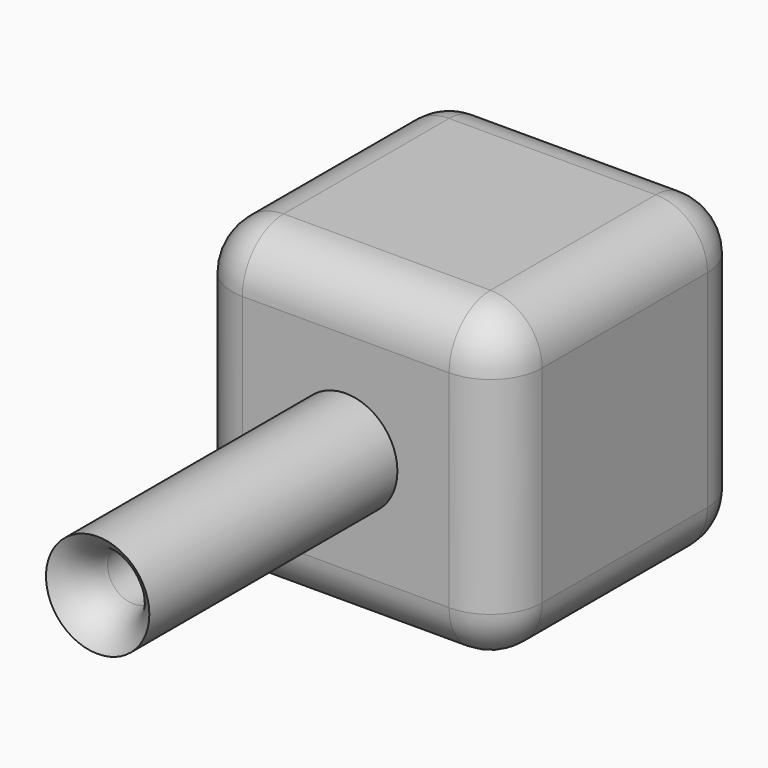
from build123d import *

# Parameters (mm, degrees)
F0_W         = 30
F0_H         = 30
F1_DEPTH     = 30
F2_R         = 5
F3_DEPTH     = 30
F4_R         = 2.5001325449
F5_DEPTH     = 60.001
F6_T1_DEPTH  = 20
F6_T3_DEPTH  = 20
F6_T5_DEPTH  = 20
F6_S9_W      = 5.1
F6_S9_H      = 5.1
F6_T10_DEPTH = 5.1
F6_S15_W     = 5.1
F6_S15_H     = 5.1
F6_T16_DEPTH = 5.1
F6_S21_W     = 5.1
F6_S21_H     = 5.1
F6_T22_DEPTH = 5.1
F6_S27_W     = 5.1
F6_S27_H     = 5.1
F6_T28_DEPTH = 5.1
F6_S33_W     = 5.1
F6_S33_H     = 5.1
F6_T34_DEPTH = 5.1
F6_S39_W     = 5.1
F6_S39_H     = 5.1
F6_T40_DEPTH = 5.1
F6_S45_W     = 5.1
F6_S45_H     = 5.1
F6_T46_DEPTH = 5.1
F6_S51_W     = 5.1
F6_S51_H     = 5.1
F6_T52_DEPTH = 5.1


# Not quite as in the source:
# - a fillet or chamfer that OpenCascade refuses, or shapes differently, is made with other operations: its cross-section is extruded or revolved along the edge and cut away or added


with BuildPart() as f1:
    # F0 (on Front) → F1 (new body)
    with BuildSketch(Plane.XZ):
        Rectangle(F0_W, F0_H)
    extrude(amount=F1_DEPTH)

    # F2 (on face) → F3 (join)
    with BuildSketch(Plane.XZ.offset(30)):
        Circle(F2_R)
    extrude(amount=F3_DEPTH)

    # F4 (on face) → F5 (cut, through all)
    with BuildSketch(Plane.XZ.offset(60)):
        Circle(F4_R)
    extrude(amount=-F5_DEPTH, mode=Mode.SUBTRACT)

    # F6: fillet of radius 5 on 13 edges, made by hand

    # F6_s2 → F6_t1 (cut)
    with BuildSketch(Plane.XZ.offset(5)):
        with BuildLine():
            ThreePointArc((10, 15), (13.5355339059, 13.5355339059), (15, 10))
            Line((15, 10), (15, 15))
            Line((15, 15), (10, 15))
        make_face()
        with BuildLine():
            ThreePointArc((-10, 15), (-13.5355339059, 13.5355339059), (-15, 10))
            Line((-15, 10), (-15, 15))
            Line((-15, 15), (-10, 15))
        make_face()
        with BuildLine():
            ThreePointArc((-15, -10), (-13.5355339059, -13.5355339059), (-10, -15))
            Line((-10, -15), (-15, -15))
            Line((-15, -15), (-15, -10))
        make_face()
        with BuildLine():
            ThreePointArc((15, -10), (13.5355339059, -13.5355339059), (10, -15))
            Line((10, -15), (15, -15))
            Line((15, -15), (15, -10))
        make_face()
    extrude(amount=F6_T1_DEPTH, mode=Mode.SUBTRACT)

    # F6_s4 → F6_t3 (cut)
    with BuildSketch(Plane.YZ.offset(-10)):
        with BuildLine():
            ThreePointArc((-25, 15), (-28.5355339059, 13.5355339059), (-30, 10))
            Line((-30, 10), (-30, 15))
            Line((-30, 15), (-25, 15))
        make_face()
        with BuildLine():
            ThreePointArc((-5, 15), (-1.4644660941, 13.5355339059), (0, 10))
            Line((0, 10), (0, 15))
            Line((0, 15), (-5, 15))
        make_face()
        with BuildLine():
            ThreePointArc((-30, -10), (-28.5355339059, -13.5355339059), (-25, -15))
            Line((-25, -15), (-30, -15))
            Line((-30, -15), (-30, -10))
        make_face()
        with BuildLine():
            ThreePointArc((0, -10), (-1.4644660941, -13.5355339059), (-5, -15))
            Line((-5, -15), (0, -15))
            Line((0, -15), (0, -10))
        make_face()
    extrude(amount=F6_T3_DEPTH, mode=Mode.SUBTRACT)

    # F6_s6 → F6_t5 (cut)
    with BuildSketch(Plane.XY.offset(-10)):
        with BuildLine():
            ThreePointArc((-15, -5), (-13.5355339059, -1.4644660941), (-10, 0))
            Line((-10, 0), (-15, 0))
            Line((-15, 0), (-15, -5))
        make_face()
        with BuildLine():
            ThreePointArc((-15, -25), (-13.5355339059, -28.5355339059), (-10, -30))
            Line((-10, -30), (-15, -30))
            Line((-15, -30), (-15, -25))
        make_face()
        with BuildLine():
            ThreePointArc((15, -5), (13.5355339059, -1.4644660941), (10, 0))
            Line((10, 0), (15, 0))
            Line((15, 0), (15, -5))
        make_face()
        with BuildLine():
            ThreePointArc((15, -25), (13.5355339059, -28.5355339059), (10, -30))
            Line((10, -30), (15, -30))
            Line((15, -30), (15, -25))
        make_face()
    extrude(amount=F6_T5_DEPTH, mode=Mode.SUBTRACT)


with BuildPart() as f6_tool8:
    # F6_s9 → F6_t10 (new body)
    with BuildSketch(Plane.XY.offset(10)):
        with Locations((12.55, -2.45)):
            Rectangle(F6_S9_W, F6_S9_H)
    extrude(amount=F6_T10_DEPTH)

    # F6_s11 → F6_t12 (revolve, cut)
    with BuildSketch(Plane(origin=(10, -5, 10), x_dir=(-0.7071067812, -0.7071067812, 0), z_dir=(-0.7071067812, 0.7071067812, 0))):
        with BuildLine():
            ThreePointArc((0, -5), (5, 0), (0, 5))
            Line((0, 5), (0, -5))
        make_face()
    revolve(axis=Axis((10, -5, 10), (0, 0, 1)), mode=Mode.SUBTRACT)


with BuildPart() as f1_1:
    add(f1.part)

    # F6_t7: cut F6_tool8
    add(f6_tool8.part, mode=Mode.SUBTRACT)


with BuildPart() as f6_tool14:
    # F6_s15 → F6_t16 (new body)
    with BuildSketch(Plane.XY.offset(10)):
        with Locations((12.55, -27.55)):
            Rectangle(F6_S15_W, F6_S15_H)
    extrude(amount=F6_T16_DEPTH)

    # F6_s17 → F6_t18 (revolve, cut)
    with BuildSketch(Plane(origin=(10, -25, 10), x_dir=(-0.7071067812, 0.7071067812, 0), z_dir=(0.7071067812, 0.7071067812, 0))):
        with BuildLine():
            ThreePointArc((0, -5), (5, 0), (0, 5))
            Line((0, 5), (0, -5))
        make_face()
    revolve(axis=Axis((10, -25, 10), (0, 0, 1)), mode=Mode.SUBTRACT)


with BuildPart() as f1_2:
    add(f1_1.part)

    # F6_t13: cut F6_tool14
    add(f6_tool14.part, mode=Mode.SUBTRACT)


with BuildPart() as f6_tool20:
    # F6_s21 → F6_t22 (new body)
    with BuildSketch(Plane.XY.offset(10)):
        with Locations((-12.55, -2.45)):
            Rectangle(F6_S21_W, F6_S21_H)
    extrude(amount=F6_T22_DEPTH)

    # F6_s23 → F6_t24 (revolve, cut)
    with BuildSketch(Plane(origin=(-10, -5, 10), x_dir=(0.7071067812, -0.7071067812, 0), z_dir=(-0.7071067812, -0.7071067812, 0))):
        with BuildLine():
            ThreePointArc((0, -5), (5, 0), (0, 5))
            Line((0, 5), (0, -5))
        make_face()
    revolve(axis=Axis((-10, -5, 10), (0, 0, 1)), mode=Mode.SUBTRACT)


with BuildPart() as f1_3:
    add(f1_2.part)

    # F6_t19: cut F6_tool20
    add(f6_tool20.part, mode=Mode.SUBTRACT)


with BuildPart() as f6_tool26:
    # F6_s27 → F6_t28 (new body)
    with BuildSketch(Plane.XY.offset(10)):
        with Locations((-12.55, -27.55)):
            Rectangle(F6_S27_W, F6_S27_H)
    extrude(amount=F6_T28_DEPTH)

    # F6_s29 → F6_t30 (revolve, cut)
    with BuildSketch(Plane(origin=(-10, -25, 10), x_dir=(0.7071067812, 0.7071067812, 0), z_dir=(0.7071067812, -0.7071067812, 0))):
        with BuildLine():
            ThreePointArc((0, -5), (5, 0), (0, 5))
            Line((0, 5), (0, -5))
        make_face()
    revolve(axis=Axis((-10, -25, 10), (0, 0, 1)), mode=Mode.SUBTRACT)


with BuildPart() as f1_4:
    add(f1_3.part)

    # F6_t25: cut F6_tool26
    add(f6_tool26.part, mode=Mode.SUBTRACT)


with BuildPart() as f6_tool32:
    # F6_s33 → F6_t34 (new body)
    with BuildSketch(Plane.YZ.offset(-10)):
        with Locations((-27.55, -12.55)):
            Rectangle(F6_S33_W, F6_S33_H)
    extrude(amount=-F6_T34_DEPTH)

    # F6_s35 → F6_t36 (revolve, cut)
    with BuildSketch(Plane(origin=(-10, -25, -10), x_dir=(0, 0.7071067812, 0.7071067812), z_dir=(0, -0.7071067812, 0.7071067812))):
        with BuildLine():
            ThreePointArc((0, -5), (5, 0), (0, 5))
            Line((0, 5), (0, -5))
        make_face()
    revolve(axis=Axis((-10, -25, -10), (-1, 0, 0)), mode=Mode.SUBTRACT)


with BuildPart() as f1_5:
    add(f1_4.part)

    # F6_t31: cut F6_tool32
    add(f6_tool32.part, mode=Mode.SUBTRACT)


with BuildPart() as f6_tool38:
    # F6_s39 → F6_t40 (new body)
    with BuildSketch(Plane.YZ.offset(10)):
        with Locations((-27.55, -12.55)):
            Rectangle(F6_S39_W, F6_S39_H)
    extrude(amount=F6_T40_DEPTH)

    # F6_s41 → F6_t42 (revolve, cut)
    with BuildSketch(Plane(origin=(10, -25, -10), x_dir=(0, 0.7071067812, 0.7071067812), z_dir=(0, 0.7071067812, -0.7071067812))):
        with BuildLine():
            ThreePointArc((0, -5), (5, 0), (0, 5))
            Line((0, 5), (0, -5))
        make_face()
    revolve(axis=Axis((10, -25, -10), (1, 0, 0)), mode=Mode.SUBTRACT)


with BuildPart() as f1_6:
    add(f1_5.part)

    # F6_t37: cut F6_tool38
    add(f6_tool38.part, mode=Mode.SUBTRACT)


with BuildPart() as f6_tool44:
    # F6_s45 → F6_t46 (new body)
    with BuildSketch(Plane.YZ.offset(-10)):
        with Locations((-2.45, -12.55)):
            Rectangle(F6_S45_W, F6_S45_H)
    extrude(amount=-F6_T46_DEPTH)

    # F6_s47 → F6_t48 (revolve, cut)
    with BuildSketch(Plane(origin=(-10, -5, -10), x_dir=(0, -0.7071067812, 0.7071067812), z_dir=(0, -0.7071067812, -0.7071067812))):
        with BuildLine():
            ThreePointArc((0, -5), (5, 0), (0, 5))
            Line((0, 5), (0, -5))
        make_face()
    revolve(axis=Axis((-10, -5, -10), (-1, 0, 0)), mode=Mode.SUBTRACT)


with BuildPart() as f1_7:
    add(f1_6.part)

    # F6_t43: cut F6_tool44
    add(f6_tool44.part, mode=Mode.SUBTRACT)


with BuildPart() as f6_tool50:
    # F6_s51 → F6_t52 (new body)
    with BuildSketch(Plane.YZ.offset(10)):
        with Locations((-2.45, -12.55)):
            Rectangle(F6_S51_W, F6_S51_H)
    extrude(amount=F6_T52_DEPTH)

    # F6_s53 → F6_t54 (revolve, cut)
    with BuildSketch(Plane(origin=(10, -5, -10), x_dir=(0, -0.7071067812, 0.7071067812), z_dir=(0, 0.7071067812, 0.7071067812))):
        with BuildLine():
            ThreePointArc((0, -5), (5, 0), (0, 5))
            Line((0, 5), (0, -5))
        make_face()
    revolve(axis=Axis((10, -5, -10), (1, 0, 0)), mode=Mode.SUBTRACT)


with BuildPart() as f1_8:
    add(f1_7.part)

    # F6_t49: cut F6_tool50
    add(f6_tool50.part, mode=Mode.SUBTRACT)

    # F6_s55 → F6_t56 (revolve, cut)
    with BuildSketch(Plane.XY):
        with BuildLine():
            ThreePointArc((2.5001325449, -55.6699495086), (3.1699672637, -58.1698832353), (5, -60))
            Line((5, -60), (2.5001325449, -60))
            Line((2.5001325449, -60), (2.5001325449, -55.6699495086))
        make_face()
    revolve(axis=Axis((0, -60, 0), (0, -1, 0)), mode=Mode.SUBTRACT)


solid = f1_8.part
